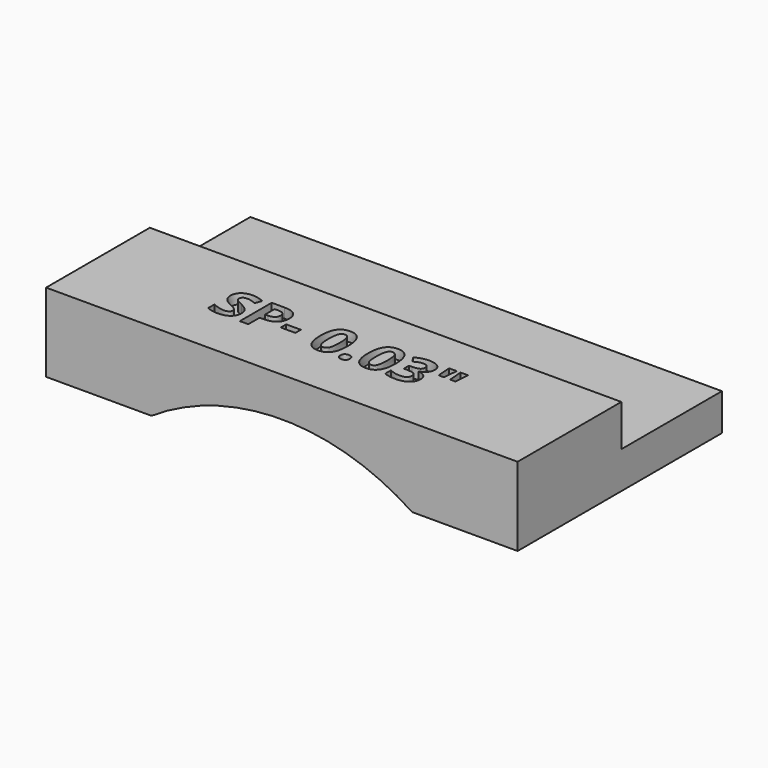
from build123d import *

# Parameters (mm, degrees)
F1_DEPTH     = 39.6875
F2_W         = 152.4
F2_H         = 25.4
F3_DEPTH     = 42.8625
F4_W         = 152.4
F4_H         = 13.462
F5_DEPTH     = 40.64
F6_TEXT_SIZE = 18.0148498393
F7_DEPTH     = 3.175


# Not quite as in the source:
# - Text() gives the source's letters only with a copy of the font that has no kerning and outlines rounded to 1/6400 em; it was checked with that copy


with BuildPart() as f1:
    # F0 (on Front) → F1 (new body)
    with BuildSketch(Plane.XZ):
        with BuildLine():
            Line((0, 25.4), (0, 0))
            Line((0, 0), (34.0788651625, 0))
            ThreePointArc((34.0788651625, 0), (76.2, 12.7), (118.3211348375, 0))
            Line((118.3211348375, 0), (152.4, 0))
            Line((152.4, 0), (152.4, 25.4))
            Line((152.4, 25.4), (0, 25.4))
        make_face()
    extrude(amount=F1_DEPTH)

    # F2 (on face) → F3 (join)
    with BuildSketch(Plane(origin=(0, 0, 0), x_dir=(-1, 0, 0), z_dir=(0, 1, 0))):
        with Locations((-76.2, 12.7)):
            Rectangle(F2_W, F2_H)
    extrude(amount=F3_DEPTH)

    # F4 (on face) → F5 (cut)
    with BuildSketch(Plane(origin=(0, 42.8625, 0), x_dir=(-1, 0, 0), z_dir=(0, 1, 0))):
        with Locations((-76.2, 18.669)):
            Rectangle(F4_W, F4_H)
    extrude(amount=-F5_DEPTH, mode=Mode.SUBTRACT)

    # F6 (on face) → F7 (cut)
    with BuildSketch(Plane.XY.offset(25.4)):
        with Locations((38.1, -23.4481918843)):
            Text('SP- 0.03"', F6_TEXT_SIZE, font='Open Sans', font_style=FontStyle.BOLD, text_align=(TextAlign.LEFT, TextAlign.BOTTOM))
    extrude(amount=-F7_DEPTH, mode=Mode.SUBTRACT)


solid = f1.part
